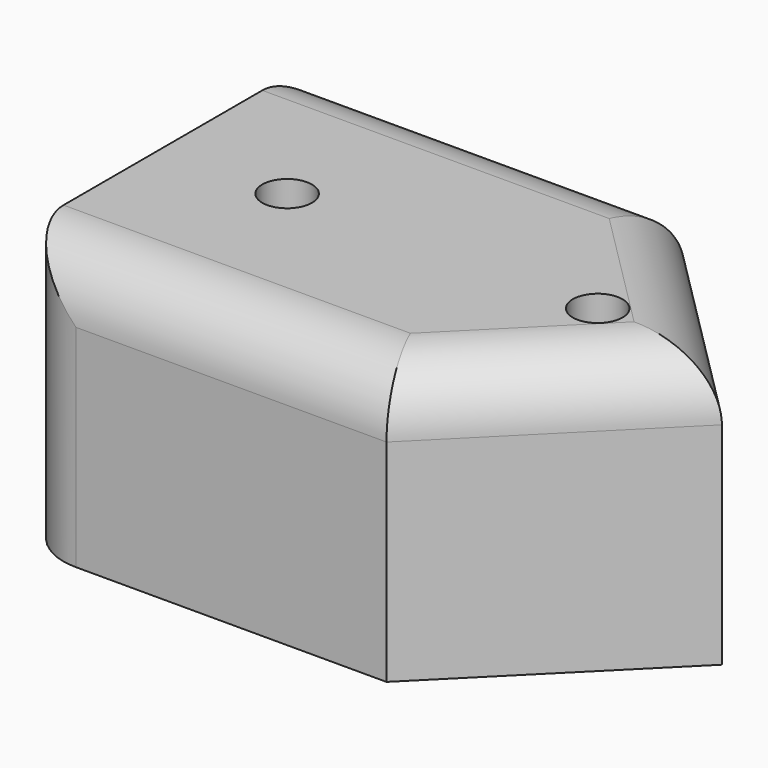
from build123d import *

# Parameters (mm, degrees)
F1_DEPTH = 22
F2_D     = 4
F3_T     = -2.5
F5_D     = 4
F5_DEPTH = 6
F5_TIP   = 1.2017212381
F6_R     = 4.99999


# Not quite as in the source:
# - a fillet or chamfer is up to 0.001 mm smaller than in the source, because OpenCascade refuses the exact size


with BuildPart() as f1:
    # F0 (on Top) → F1 (new body)
    with BuildSketch(Plane.XY):
        Polygon((-15, -15), (0, 0), (-15, 15), (-45, 15), (-45, -15), align=None)
    extrude(amount=F1_DEPTH)

    # F2 (through all)
    with Locations(Plane(origin=(0, 0, 0), x_dir=(1, 0, 0), z_dir=(0, 0, -1))):
        with Locations((-35, 0), (-10, 0)):
            Hole(F2_D / 2)

    # F3
    f3_openings = [f1.faces().sort_by_distance(p)[0] for p in [
        (-26.079977, 0, 0),
    ]]
    offset(amount=F3_T, openings=f3_openings)

    # F5
    with Locations(Plane(origin=(-45, 0, 0), x_dir=(0, -1, 0), z_dir=(-1, 0, 0))):
        with Locations((-8, 11), (8, 11)):
            Hole(F5_D / 2, depth=F5_DEPTH)
            with Locations((0, 0, -(F5_DEPTH + F5_TIP / 2))):  # 118° drill point
                Cone(0, F5_D / 2, F5_TIP, mode=Mode.SUBTRACT)

    # F6 (radius 5 in the source; OpenCascade refuses exactly that, so slightly less here)
    f6_edges = [f1.edges().sort_by_distance(p)[0] for p in [
        (-30, -15, 22),
        (-7.5, -7.5, 22),
        (-7.5, 7.5, 22),
        (-30, 15, 22),
        (-45, 15, 11),
        (-45, -15, 11),
    ]]
    fillet(f6_edges, radius=F6_R)


solid = f1.part
